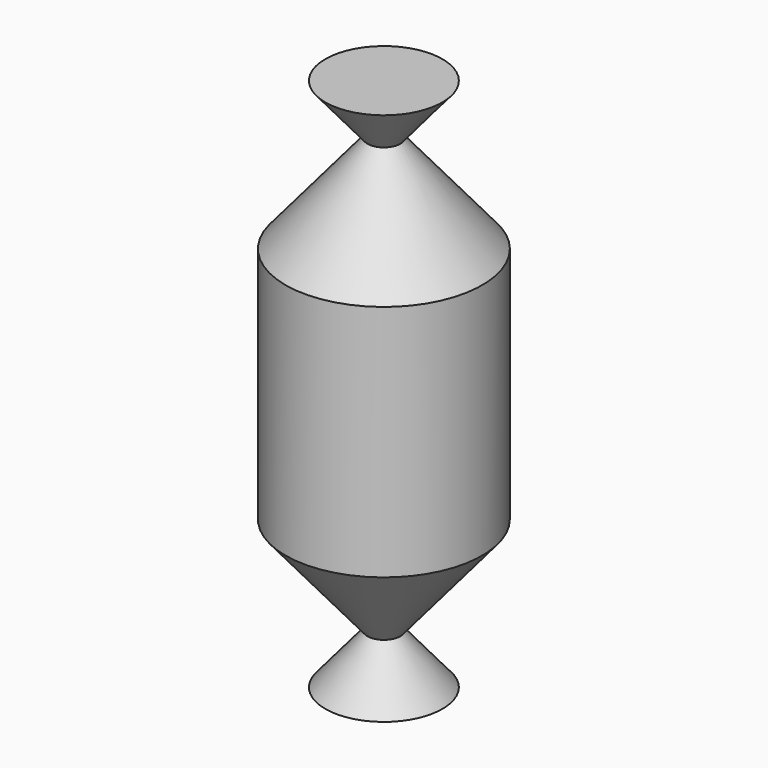
from build123d import *


# Not quite as in the source:
# - a feature of the source that left no trace in its solid (it failed there, or was rolled back) is left out


with BuildPart() as f1:
    # F0 (on Front) → F1 (revolve)
    with BuildSketch(Plane.XZ):
        Polygon((-38.1, 46.1013156182), (-38.1, 0), (-38.1, -46.1013156182), (-6.35, -83.9394921831), (0, -91.5071274961), (0, 83.9394921831), (-6.35, 83.9394921831), align=None)
        Polygon((-22.676805286, 103.3970210383), (-6.35, 83.9394921831), (0, 91.5071274961), (0, 103.3970210383), align=None)
        Polygon((0, 91.5071274961), (-6.35, 83.9394921831), (0, 83.9394921831), align=None)
        Polygon((0, -91.5071274961), (-6.35, -83.9394921831), (-22.676805286, -103.3970210383), (0, -103.3970210383), align=None)
    revolve(axis=Axis((0, 0, 0), (0, 0, -1)))


solid = f1.part
